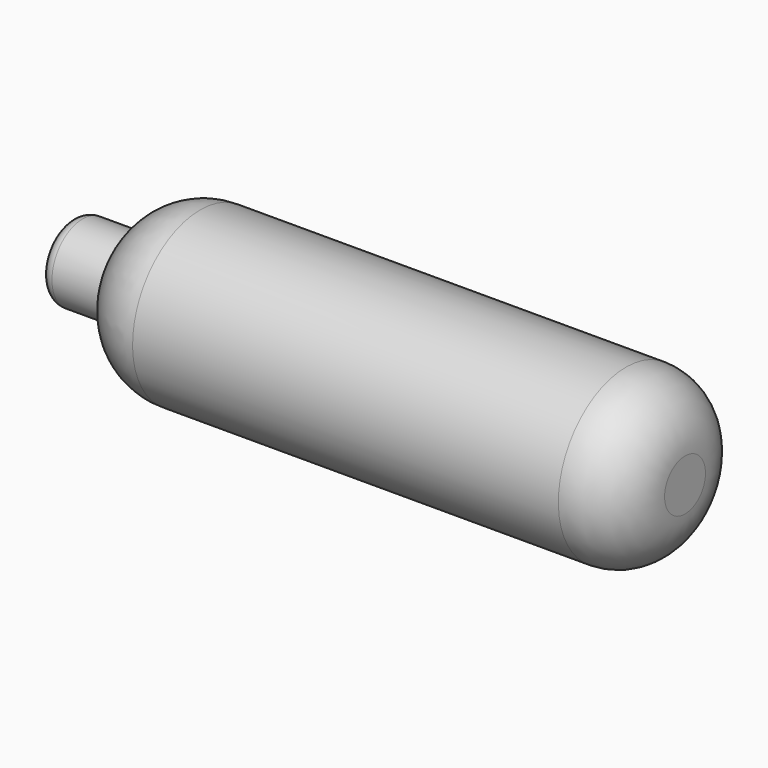
from build123d import *

# Parameters (mm, degrees)
F2_R = 6.096
F4_R = 1.27


# Not quite as in the source:
# - a fillet or chamfer that OpenCascade refuses, or shapes differently, is made with other operations: its cross-section is extruded or revolved along the edge and cut away or added


with BuildPart() as f1:
    # F0 (on Front) → F1 (revolve)
    with BuildSketch(Plane.XZ):
        Polygon((38.2069466584, 0), (38.2069466584, 8.7376), (-18.9430533416, 8.7376), (-18.9430533416, 3.9624), (-25.2930533416, 3.9624), (-25.2930533416, 0), align=None)
    revolve(axis=Axis((6.4569466584, 0, 0), (-1, 0, 0)))

    # F2
    f2_edges = [f1.edges().sort_by_distance(p)[0] for p in [
        (38.206947, 0, -8.7376),
    ]]
    fillet(f2_edges, radius=F2_R)

    # F3: fillet of radius 7.62 on 1 edges, made by hand

    # F3_s1 → F3_t2 (revolve, cut)
    with BuildSketch(Plane.XZ):
        with BuildLine():
            ThreePointArc((-11.8740001546, 8.7376), (-16.139385483, 7.4319398705), (-18.9430533416, 3.9624))
            Line((-18.9430533416, 3.9624), (-18.9430533416, 8.7376))
            Line((-18.9430533416, 8.7376), (-11.8740001546, 8.7376))
        make_face()
    revolve(axis=Axis((-18.9430533416, 0, 0), (-1, 0, 0)), mode=Mode.SUBTRACT)

    # F4
    f4_edges = [f1.edges().sort_by_distance(p)[0] for p in [
        (-25.293053, 0, -3.9624),
    ]]
    fillet(f4_edges, radius=F4_R)


solid = f1.part
